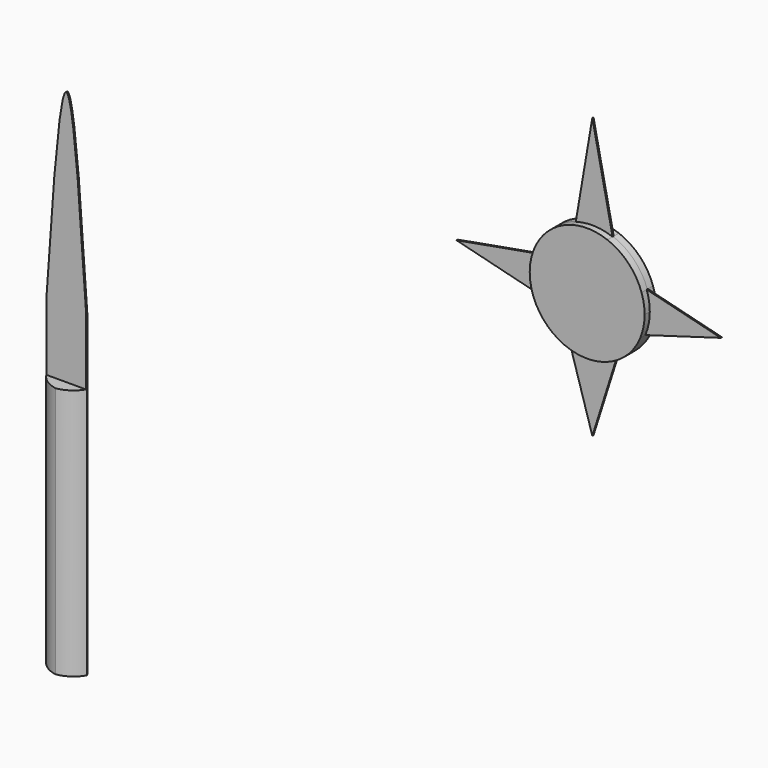
from build123d import *

# Parameters (mm, degrees)
F1_DEPTH    = 0.127
F2_DEPTH    = 2.54
F3_T1_DEPTH = 69.9690318011
F5_DEPTH    = 1.27
F6_DEPTH    = 0.127


# Not quite as in the source:
# - a fillet or chamfer that OpenCascade refuses, or shapes differently, is made with other operations: its cross-section is extruded or revolved along the edge and cut away or added


with BuildPart() as f1:
    # F0 (on Front) → F1 (new body, symmetric)
    with BuildSketch(Plane.XZ):
        with BuildLine():
            add(Edge.make_bspline(
                [(-61.6640038788, -4.5790136792), (-60.2394230664, 18.0107697379), (-57.3902614415, 63.190336572), (-54.5410998166, 18.0107697379), (-53.1165190041, -4.5790136792)],
                knots=[0, 0, 0, 0, 0.5, 1, 1, 1, 1], degree=3))
            Line((-61.6640038788, -4.5790136792), (-53.1165190041, -4.5790136792))
        make_face()
    extrude(amount=F1_DEPTH, both=True)

    # F0 (on Front) → F2 (join, symmetric)
    with BuildSketch(Plane.XZ):
        Polygon((-61.6640038788, -4.5790136792), (-53.1165190041, -8.8321231306), (-53.1165190041, -4.5790136792), align=None)
        Polygon((-61.6640038788, -4.5790136792), (-61.6640038788, -12.8659997135), (-53.1165190041, -8.8321231306), align=None)
        Polygon((-61.6640038788, -12.8659997135), (-53.1165190041, -15.6753063202), (-53.1165190041, -8.8321231306), align=None)
        Polygon((-61.6640038788, -12.8659997135), (-61.6640038788, -19.7091810405), (-53.1165190041, -15.6753063202), align=None)
        Polygon((-61.6640038788, -19.7091810405), (-53.1165190041, -23.5269572586), (-53.1165190041, -15.6753063202), align=None)
        Polygon((-61.6640038788, -19.7091810405), (-61.6640038788, -27.4887997657), (-53.1165190041, -23.5269572586), align=None)
        Polygon((-61.6640038788, -27.4887997657), (-53.1165190041, -31.4506441355), (-53.1165190041, -23.5269572586), align=None)
        Polygon((-61.6640038788, -27.4887997657), (-61.6640038788, -37.051204592), (-53.1165190041, -31.4506441355), align=None)
        Polygon((-61.6640038788, -37.051204592), (-53.1165190041, -41.0130489618), (-53.1165190041, -31.4506441355), align=None)
        Polygon((-61.6640038788, -37.051204592), (-61.6640038788, -44.6657761931), (-53.1165190041, -41.0130489618), align=None)
        Polygon((-61.6640038788, -44.6657761931), (-53.1165190041, -49.1480454803), (-53.1165190041, -41.0130489618), align=None)
        Polygon((-61.6640038788, -44.6657761931), (-61.6640038788, -49.1480454803), (-53.1165190041, -49.1480454803), align=None)
    extrude(amount=F2_DEPTH, both=True)

    # F3: fillet of radius 5.08 on 4 edges, made by hand

    # F3_s2 → F3_t1 (cut)
    with BuildSketch(Plane.XY.offset(-61.8480454803)):
        with BuildLine():
            ThreePointArc((-61.6640038788, -2.54), (-60.1761063273, 1.0521024484), (-56.5840038788, 2.54))
            Line((-56.5840038788, 2.54), (-61.6640038788, 2.54))
            Line((-61.6640038788, 2.54), (-61.6640038788, -2.54))
        make_face()
        with BuildLine():
            ThreePointArc((-61.6640038788, 2.54), (-60.1761063273, -1.0521024484), (-56.5840038788, -2.54))
            Line((-56.5840038788, -2.54), (-61.6640038788, -2.54))
            Line((-61.6640038788, -2.54), (-61.6640038788, 2.54))
        make_face()
        with BuildLine():
            ThreePointArc((-53.1165190041, 2.54), (-54.6044165557, -1.0521024484), (-58.1965190041, -2.54))
            Line((-58.1965190041, -2.54), (-53.1165190041, -2.54))
            Line((-53.1165190041, -2.54), (-53.1165190041, 2.54))
        make_face()
        with BuildLine():
            ThreePointArc((-53.1165190041, -2.54), (-54.6044165557, 1.0521024484), (-58.1965190041, 2.54))
            Line((-58.1965190041, 2.54), (-53.1165190041, 2.54))
            Line((-53.1165190041, 2.54), (-53.1165190041, -2.54))
        make_face()
    extrude(amount=F3_T1_DEPTH, mode=Mode.SUBTRACT)


with BuildPart() as f5:
    # F4 (on Front) → F5 (new body, symmetric)
    with BuildSketch(Plane.XZ):
        with BuildLine():
            ThreePointArc((45.1031894134, 36.0872628929), (45.6855333143, 38.000150468), (45.8821839732, 39.9900227785))
            ThreePointArc((45.8821839732, 39.9900227785), (45.7462436924, 41.6469572454), (45.3420584857, 43.2595780645))
            ThreePointArc((45.3420584857, 43.2595780645), (43.0213801023, 47.0597550319), (39.2992154724, 49.5036011011))
            ThreePointArc((39.2992154724, 49.5036011011), (36.0610548886, 50.1500782492), (32.7865184008, 49.7246050309))
            ThreePointArc((32.7865184008, 49.7246050309), (28.3890172345, 47.0367817513), (25.8748064715, 42.5377646665))
            ThreePointArc((25.8748064715, 42.5377646665), (25.566561341, 39.416611169), (26.2243841751, 36.3500359891))
            ThreePointArc((26.2243841751, 36.3500359891), (28.3751844661, 32.9576755169), (31.672057957, 30.6631871971))
            ThreePointArc((31.672057957, 30.6631871971), (35.8417057181, 29.8248929156), (39.9894001299, 30.7658131144))
            ThreePointArc((39.9894001299, 30.7658131144), (43.0462567434, 32.9460861946), (45.1031894134, 36.0872628929))
        make_face()
    extrude(amount=F5_DEPTH, both=True)

    # F4 (on Front) → F6 (join, symmetric)
    with BuildSketch(Plane.XZ):
        with BuildLine():
            ThreePointArc((26.2243841751, 36.3500359891), (25.566561341, 39.416611169), (25.8748064715, 42.5377646665))
            Line((25.8748064715, 42.5377646665), (11.667765677, 39.9900227785))
            Line((11.667765677, 39.9900227785), (26.2243841751, 36.3500359891))
        make_face()
        with BuildLine():
            ThreePointArc((32.7865184008, 49.7246050309), (36.0610548886, 50.1500782492), (39.2992154724, 49.5036011011))
            Line((39.2992154724, 49.5036011011), (35.7162803411, 66.886715591))
            Line((35.7162803411, 66.886715591), (32.7865184008, 49.7246050309))
        make_face()
        with BuildLine():
            Line((35.7162803411, 17.3209942877), (39.9894001299, 30.7658131144))
            ThreePointArc((39.9894001299, 30.7658131144), (35.8417057181, 29.8248929156), (31.672057957, 30.6631871971))
            Line((31.672057957, 30.6631871971), (35.7162803411, 17.3209942877))
        make_face()
        with BuildLine():
            ThreePointArc((45.3420584857, 43.2595780645), (45.7462436924, 41.6469572454), (45.8821839732, 39.9900227785))
            ThreePointArc((45.8821839732, 39.9900227785), (45.6855333143, 38.000150468), (45.1031894134, 36.0872628929))
            Line((45.1031894134, 36.0872628929), (58.4464035928, 39.9900227785))
            Line((58.4464035928, 39.9900227785), (45.3420584857, 43.2595780645))
        make_face()
    extrude(amount=F6_DEPTH, both=True)


solid = Compound([f1.part, f5.part])
